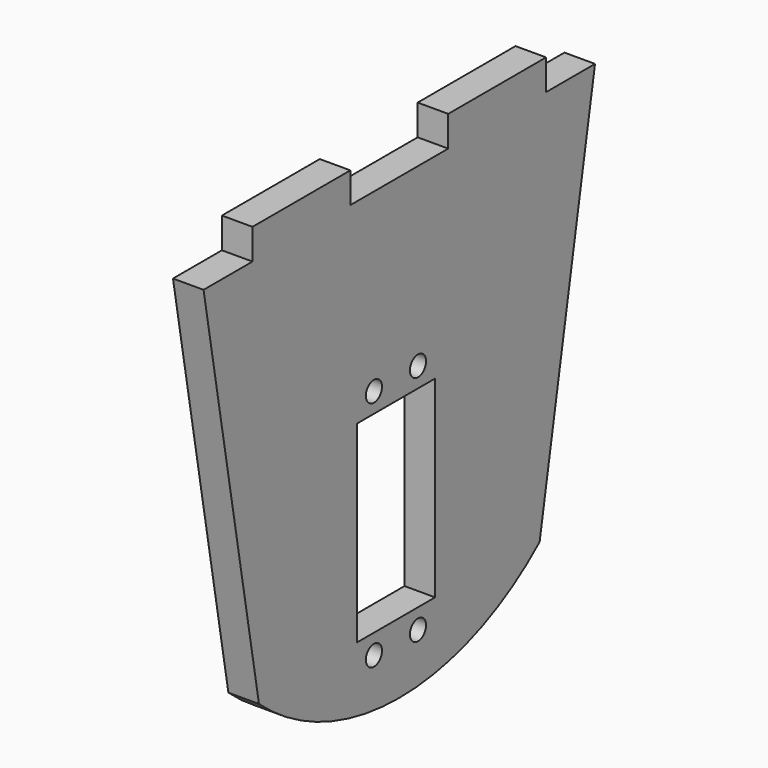
from build123d import *

# Parameters (mm, degrees)
F1_DEPTH = 6.35
F2_W     = 12.7
F2_H     = 6.35
F3_DEPTH = 25.4
F4_W     = 20.32
F4_H     = 40.005
F4_R     = 2.0955
F5_DEPTH = 25.4


# Not quite as in the source:
# - a feature names something its author has since deleted; it is built from what else it names


with BuildPart() as f1:
    # F0 (on Right) → F1 (new body)
    with BuildSketch(Plane.YZ):
        with BuildLine():
            Line((50.8, 0), (0, 0))
            Line((0, 0), (0, -6.35))
            Line((0, -6.35), (14.3783799252, -87.8938446653))
            ThreePointArc((14.3783799252, -87.8938446653), (31.3423979963, -98.0600456848), (50.8, -101.6))
            Line((50.8, -101.6), (50.8, 0))
        make_face()
        with BuildLine():
            Line((101.6, 0), (50.8, 0))
            Line((50.8, 0), (50.8, -101.6))
            ThreePointArc((50.8, -101.6), (70.2576020037, -98.0600456848), (87.2216200748, -87.8938446653))
            Line((87.2216200748, -87.8938446653), (101.6, -6.35))
            Line((101.6, -6.35), (101.6, 0))
        make_face()
    extrude(amount=F1_DEPTH)

    # F2 (on face) → F3 (cut)
    with BuildSketch(Plane.YZ.offset(6.35)):
        with Locations((95.25, -3.175)):
            Rectangle(F2_W, F2_H)
        with Locations((44.45, -3.175)):
            Rectangle(F2_W, F2_H)
        with Locations((6.35, -3.175)):
            Rectangle(F2_W, F2_H)
        with Locations((57.15, -3.175)):
            Rectangle(F2_W, F2_H)
    extrude(amount=-F3_DEPTH, mode=Mode.SUBTRACT)

    # F4 (on face) → F5 (cut)
    with BuildSketch(Plane.YZ.offset(6.35)):
        with Locations((49.9361574873, -66.9925)):
            Rectangle(F4_W, F4_H)
        with Locations((44.2211574873, -42.8625)):
            Circle(F4_R)
        with Locations((55.6511574873, -42.8625)):
            Circle(F4_R)
        with Locations((55.6511574873, -91.1225)):
            Circle(F4_R)
        with Locations((44.2211574873, -91.1225)):
            Circle(F4_R)
    extrude(amount=-F5_DEPTH, mode=Mode.SUBTRACT)


solid = f1.part
